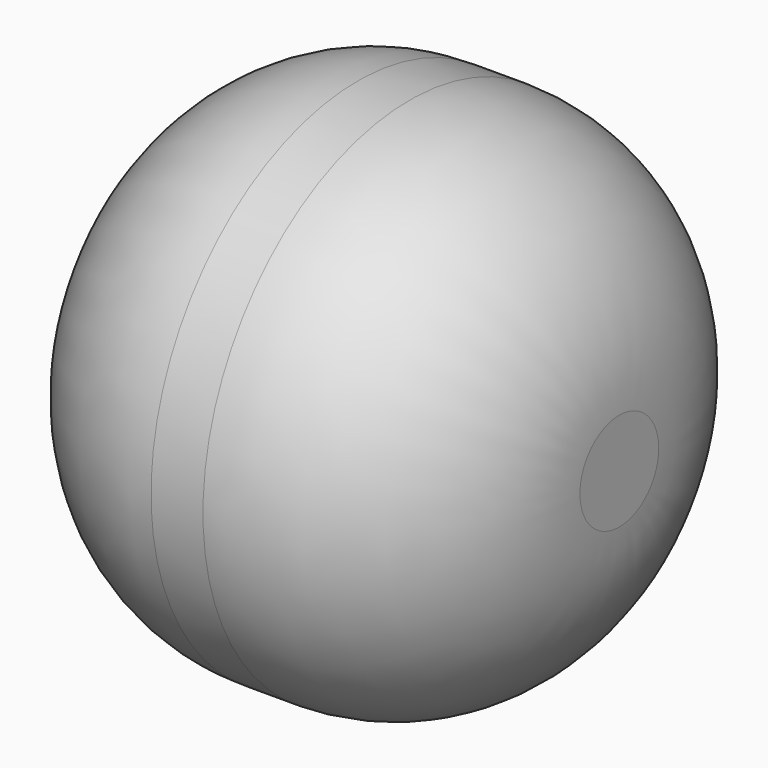
from build123d import *

# Parameters (mm, degrees)
F0_R     = 95.3421100221
F1_DEPTH = 86.7594629526
F2_R     = 77.1877360698


# Not quite as in the source:
# - the program builds the solid bodies; features that only make, move or delete a surface that nothing else refers to are left out


with BuildPart() as f1:
    # F0 (on Right) → F1 (new body, symmetric)
    with BuildSketch(Plane.YZ):
        with Locations((-1.49012e-05, 0.2395585179)):
            Circle(F0_R)
    extrude(amount=F1_DEPTH, both=True)

    # F2
    f2_edges = [f1.edges().sort_by_distance(p)[0] for p in [
        (-86.759463, -95.342125, 0.239559),
        (86.759463, -95.342125, 0.239559),
    ]]
    fillet(f2_edges, radius=F2_R)


solid = f1.part
